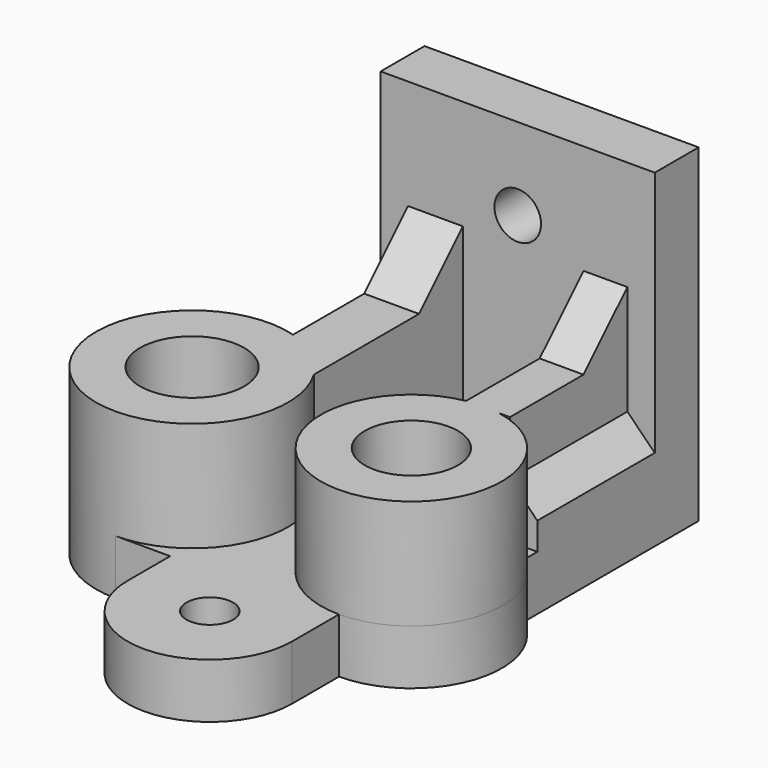
from build123d import *

# Parameters (mm, degrees)
F0_R          = 4.75
F0_R_2        = 2.125
F0_R_3        = 4.25
F1_DEPTH      = 5
F2_W          = 25
F2_H          = 5
F3_DEPTH      = 25
F4_R          = 8.75
F4_R_2        = 4.75
F4_R_3        = 8.25
F4_R_4        = 4.25
F5_DEPTH      = 10
F6_R          = 2.125
F7_DEPTH      = 5.001
F8_W          = 5
F8_H          = 16.9930609057
F8_W_2        = 4
F8_H_2        = 13.3875096302
F9_DEPTH      = 10
F10_T1_DEPTH  = 5
F10_T3_DEPTH  = 4
F10_T8_DEPTH  = 30.7168298797
F10_T13_DEPTH = 29.7168298797
F10_T18_DEPTH = 25.9731600242
F10_S20_R     = 4.75
F10_T21_DEPTH = 15
F10_T25_DEPTH = 13.3875096302


# Not quite as in the source:
# - a fillet or chamfer that OpenCascade refuses, or shapes differently, is made with other operations: its cross-section is extruded or revolved along the edge and cut away or added


with BuildPart() as f1:
    # F0 (on Top) → F1 (new body)
    with BuildSketch(Plane.XY):
        with BuildLine():
            Line((12.5, 26.5), (0, 26.5))
            Line((0, 26.5), (-12.5, 26.5))
            Line((-12.5, 26.5), (-12.5, 8.75))
            ThreePointArc((-12.5, 8.75), (-21.25, 0), (-12.5, -8.75))
            Line((-12.5, -8.75), (-7.5, -8.75))
            Line((-7.5, -8.75), (-7.5, -13.6))
            ThreePointArc((-7.5, -13.6), (-5.3033008589, -18.9033008589), (0, -21.1))
            ThreePointArc((0, -21.1), (5.3033008589, -18.9033008589), (7.5, -13.6))
            Line((7.5, -13.6), (7.5, -8.25))
            ThreePointArc((7.5, -8.25), (15.3166703137, -2.6385915194), (12.5, 6.5622023742))
            Line((12.5, 6.5622023742), (12.5, 26.5))
        make_face()
        with Locations((-12.5, 0)):
            Circle(F0_R, mode=Mode.SUBTRACT)
        with Locations((0, -13.6)):
            Circle(F0_R_2, mode=Mode.SUBTRACT)
        with Locations((7.5, 0)):
            Circle(F0_R_3, mode=Mode.SUBTRACT)
        with Locations((0, 16.5)):
            Circle(F0_R_2, mode=Mode.SUBTRACT)
    extrude(amount=F1_DEPTH)

    # F2 (on face) → F3 (join)
    with BuildSketch(Plane.XY.offset(5)):
        with Locations((0, 24)):
            Rectangle(F2_W, F2_H)
    extrude(amount=F3_DEPTH)

    # F4 (on face) → F5 (join)
    with BuildSketch(Plane.XY.offset(5)):
        with Locations((-12.5, 0)):
            Circle(F4_R)
        with Locations((-12.5, 0)):
            Circle(F4_R_2, mode=Mode.SUBTRACT)
        with Locations((7.5, 0)):
            Circle(F4_R_3)
        with Locations((7.5, 0)):
            Circle(F4_R_4, mode=Mode.SUBTRACT)
    extrude(amount=F5_DEPTH)

    # F6 (on face) → F7 (cut, through all)
    with BuildSketch(Plane.XZ.offset(-21.5)):
        with Locations((0, 22.5)):
            Circle(F6_R)
    extrude(amount=-F7_DEPTH, mode=Mode.SUBTRACT)

    # F8 (on face) → F9 (join)
    with BuildSketch(Plane.XY.offset(5)):
        with Locations((-7.5, 13.0034695472)):
            Rectangle(F8_W, F8_H)
        with Locations((8, 14.8062451849)):
            Rectangle(F8_W_2, F8_H_2)
    extrude(amount=F9_DEPTH)

    # F10: chamfer of 5 on 4 edges, made by hand

    # F10_s2 → F10_t1 (join)
    with BuildSketch(Plane.YZ.offset(-10)):
        Polygon((16.5, 15), (21.5, 20), (21.5, 15), align=None)
    extrude(amount=F10_T1_DEPTH)

    # F10_s4 → F10_t3 (join)
    with BuildSketch(Plane.YZ.offset(6)):
        Polygon((21.5, 20), (16.5, 15), (21.5, 15), align=None)
    extrude(amount=F10_T3_DEPTH)


with BuildPart() as f10_tool6:
    # F10_s7 → F10_t8 (new body)
    with BuildSketch(Plane.YZ.offset(7.8584149398)):
        Polygon((16.5, 15), (21.5, 20), (21.5, 15), align=None)
    extrude(amount=-F10_T8_DEPTH)

    split(bisect_by=Plane.YZ.offset(6), keep=Keep.TOP)


with BuildPart() as f1_1:
    add(f1.part)

    # F10_t5: union F10_tool6
    add(f10_tool6.part)


with BuildPart() as f10_tool11:
    # F10_s12 → F10_t13 (new body)
    with BuildSketch(Plane.YZ.offset(22.8584149398)):
        Polygon((21.5, 20), (16.5, 15), (21.5, 15), align=None)
    extrude(amount=-F10_T13_DEPTH)

    split(bisect_by=Plane.YZ.offset(-5), keep=Keep.BOTTOM)


with BuildPart() as f1_2:
    add(f1_1.part)

    # F10_t10: union F10_tool11
    add(f10_tool11.part)


with BuildPart() as f10_tool16:
    # F10_s17 → F10_t18 (new body)
    with BuildSketch(Plane.XZ.offset(-21.5)):
        Polygon((-10, 10), (-15, 5), (-10, 5), align=None)
    extrude(amount=F10_T18_DEPTH)

    split(bisect_by=Plane.YZ.offset(-12.5), keep=Keep.TOP)

    # F10_s20 → F10_t21 (cut, symmetric)
    with BuildSketch(Plane.XY.offset(7.5)):
        with Locations((-12.5, 0)):
            Circle(F10_S20_R)
    extrude(amount=F10_T21_DEPTH, both=True, mode=Mode.SUBTRACT)


with BuildPart() as f1_3:
    add(f1_2.part)

    # F10_t15: union F10_tool16
    add(f10_tool16.part)


with BuildPart() as f10_tool23:
    # F10_s24 → F10_t25 (new body)
    with BuildSketch(Plane.XZ.offset(-8.1124903698)):
        Polygon((10, 10), (15, 5), (10, 5), align=None)
    extrude(amount=-F10_T25_DEPTH)

    split(bisect_by=Plane.YZ.offset(12.5), keep=Keep.BOTTOM)


with BuildPart() as f1_4:
    add(f1_3.part)

    # F10_t22: union F10_tool23
    add(f10_tool23.part)


solid = f1_4.part
